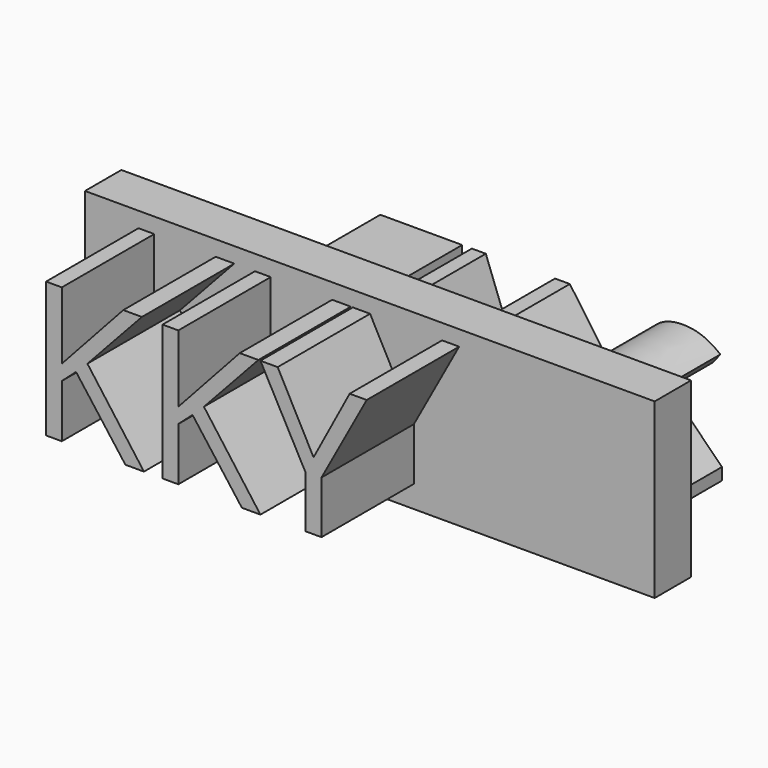
from build123d import *

# Parameters (mm, degrees)
F0_W         = 125.2691149712
F0_H         = 38.0692742765
F1_DEPTH     = 10
F3_TEXT_SIZE = 41.7358888727
F4_DEPTH     = 25.4
F5_TEXT_SIZE = 37.8863691973
F6_DEPTH     = 20


# Not quite as in the source:
# - Text() gives the source's letters only with a copy of the font that has no kerning and outlines rounded to 1/6400 em; it was checked with that copy


with BuildPart() as f1:
    # F0 (on Front) → F1 (new body)
    with BuildSketch(Plane.XZ):
        with Locations((62.6345574856, 19.0346371382)):
            Rectangle(F0_W, F0_H)
    extrude(amount=F1_DEPTH)

    # F3 (on face) → F4 (join)
    with BuildSketch(Plane.XZ.offset(10)):
        with Locations((7.6660891064, 4.8854034394)):
            Text('KKY', F3_TEXT_SIZE, font='Open Sans', text_align=(TextAlign.LEFT, TextAlign.BOTTOM))
    extrude(amount=F4_DEPTH)

    # F5 (on face) → F6 (join)
    with BuildSketch(Plane(origin=(0, 0, 0), x_dir=(-1, 0, 0), z_dir=(0, 1, 0))):
        with Locations((-117.9087013006, 7.5354417786)):
            Text('24/7', F5_TEXT_SIZE, font='Open Sans', text_align=(TextAlign.LEFT, TextAlign.BOTTOM))
    extrude(amount=F6_DEPTH)


solid = f1.part
